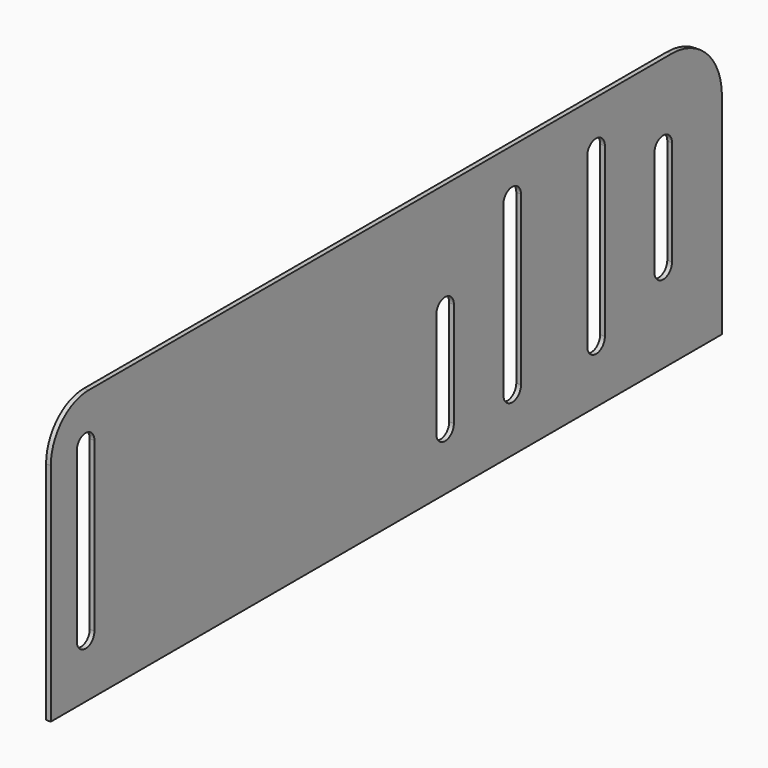
from build123d import *

# Parameters (mm, degrees)
F1_DEPTH = 4.5


# Not quite as in the source:
# - a feature names something its author has since deleted; it is built from what else it names


with BuildPart() as f1:
    # F0 (on Right) → F1 (new body)
    with BuildSketch(Plane.YZ):
        with BuildLine():
            Line((-100, -666.4014723765), (294.8394132124, -666.4014723765))
            Line((294.8394132124, -666.4014723765), (294.8394132124, -466.4014723765))
            ThreePointArc((294.8394132124, -466.4014723765), (277.2658200836, -423.9750655053), (234.8394132124, -406.4014723765))
            Line((234.8394132124, -406.4014723765), (-460.1605867876, -406.4014723765))
            ThreePointArc((-460.1605867876, -406.4014723765), (-491.980391941, -419.5816672231), (-505.1605867876, -451.4014723765))
            Line((-505.1605867876, -451.4014723765), (-505.1605867876, -666.4014723765))
            Line((-505.1605867876, -666.4014723765), (-100, -666.4014723765))
        make_face()
        with BuildLine():
            ThreePointArc((-24.6605867876, -611.4014723765), (-35.1605867876, -621.9014723765), (-45.6605867876, -611.4014723765))
            Line((-45.6605867876, -611.4014723765), (-45.6605867876, -511.4014723765))
            ThreePointArc((-45.6605867876, -511.4014723765), (-35.1605867876, -500.9014723765), (-24.6605867876, -511.4014723765))
            Line((-24.6605867876, -511.4014723765), (-24.6605867876, -611.4014723765))
        make_face(mode=Mode.SUBTRACT)
        with BuildLine():
            ThreePointArc((-453.1605867876, -611.4014723765), (-463.6605867876, -621.9014723765), (-474.1605867876, -611.4014723765))
            Line((-474.1605867876, -611.4014723765), (-474.1605867876, -451.4014723765))
            ThreePointArc((-474.1605867876, -451.4014723765), (-463.6605867876, -440.9014723765), (-453.1605867876, -451.4014723765))
            Line((-453.1605867876, -451.4014723765), (-453.1605867876, -611.4014723765))
        make_face(mode=Mode.SUBTRACT)
        with BuildLine():
            Line((34.3394132124, -611.4014723765), (34.3394132124, -451.4014723765))
            ThreePointArc((34.3394132124, -451.4014723765), (44.8394132124, -440.9014723765), (55.3394132124, -451.4014723765))
            Line((55.3394132124, -451.4014723765), (55.3394132124, -611.4014723765))
            ThreePointArc((55.3394132124, -611.4014723765), (44.8394132124, -621.9014723765), (34.3394132124, -611.4014723765))
        make_face(mode=Mode.SUBTRACT)
        with BuildLine():
            Line((134.3394132124, -611.4014723765), (134.3394132124, -451.4014723765))
            ThreePointArc((134.3394132124, -451.4014723765), (144.8394132124, -440.9014723765), (155.3394132124, -451.4014723765))
            Line((155.3394132124, -451.4014723765), (155.3394132124, -611.4014723765))
            ThreePointArc((155.3394132124, -611.4014723765), (144.8394132124, -621.9014723765), (134.3394132124, -611.4014723765))
        make_face(mode=Mode.SUBTRACT)
        with BuildLine():
            ThreePointArc((235.3394132124, -581.4014723765), (224.8394132124, -591.9014723765), (214.3394132124, -581.4014723765))
            Line((214.3394132124, -581.4014723765), (214.3394132124, -481.4014723765))
            ThreePointArc((214.3394132124, -481.4014723765), (224.8394132124, -470.9014723765), (235.3394132124, -481.4014723765))
            Line((235.3394132124, -481.4014723765), (235.3394132124, -581.4014723765))
        make_face(mode=Mode.SUBTRACT)
    extrude(amount=F1_DEPTH)


solid = f1.part
